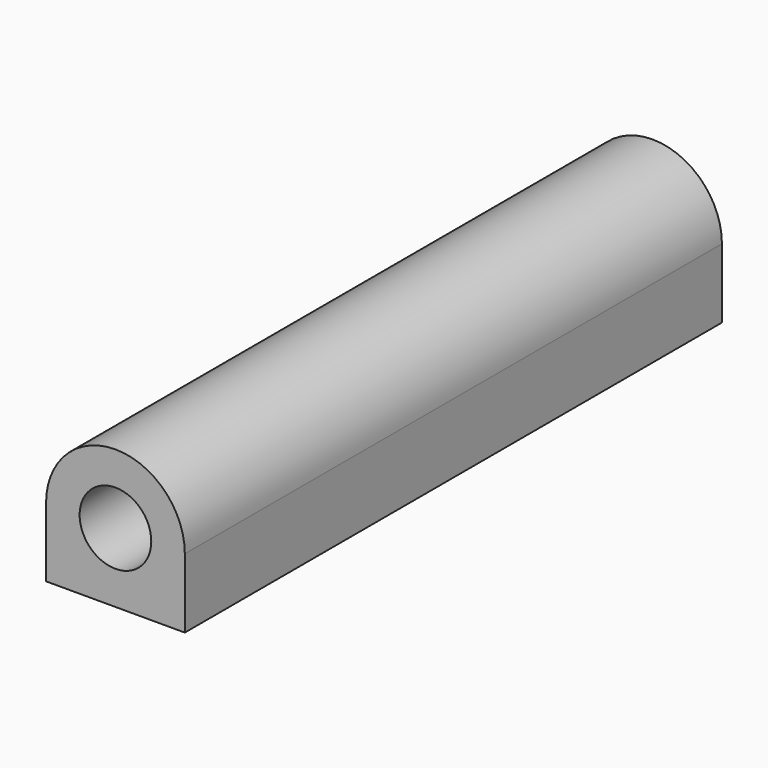
from build123d import *

# Parameters (mm, degrees)
F0_R         = 3.2
F1_DEPTH     = 30
F2_TEXT_SIZE = 11.1111111111
F3_DEPTH     = 0.6
F4_R         = 3.2
F5_DEPTH     = 2


# Not quite as in the source:
# - Text() gives the source's letters only with a copy of the font that has no kerning and outlines rounded to 1/6400 em; it was checked with that copy


with BuildPart() as f1:
    # F0 (on Front) → F1 (new body, symmetric)
    with BuildSketch(Plane.XZ):
        with BuildLine():
            ThreePointArc((0, -6.2), (4.3840620434, -4.3840620434), (6.2, 0))
            ThreePointArc((6.2, 0), (0, 6.2), (-6.2, 0))
            ThreePointArc((-6.2, 0), (-4.3840620434, -4.3840620434), (0, -6.2))
        make_face()
        Circle(F0_R, mode=Mode.SUBTRACT)
        with BuildLine():
            Line((6.2, -6.2), (6.2, 0))
            ThreePointArc((6.2, 0), (4.3840620434, -4.3840620434), (0, -6.2))
            Line((0, -6.2), (6.2, -6.2))
        make_face()
        with BuildLine():
            ThreePointArc((0, -6.2), (-4.3840620434, -4.3840620434), (-6.2, 0))
            Line((-6.2, 0), (-6.2, -6.2))
            Line((-6.2, -6.2), (0, -6.2))
        make_face()
    extrude(amount=F1_DEPTH, both=True)

    # F2 (on face) → F3 (cut)
    with BuildSketch(Plane(origin=(0, 0, -6.2), x_dir=(1, 0, 0), z_dir=(0, 0, -1))):
        with BuildLine():
            Line((1.6892361111, 11.2586805556), (1.1892361111, 11.2586805556))
            Line((1.1892361111, 11.2586805556), (1.2118055556, 10.6180555556))
            add(Edge.make_bspline(
                [(1.2118055556, 10.6180555556), (1.2326388889, 9.8958333333), (1.4713541667, 9.5434027778)],
                knots=[0, 0, 0, 1, 1, 1], degree=2))
            add(Edge.make_bspline(
                [(1.4713541667, 9.5434027778), (1.7100694444, 9.1909722222), (2.1979166667, 9.1909722222)],
                knots=[0, 0, 0, 1, 1, 1], degree=2))
            add(Edge.make_bspline(
                [(2.1979166667, 9.1909722222), (2.8993055556, 9.1909722222), (2.8993055556, 9.9930555556)],
                knots=[0, 0, 0, 1, 1, 1], degree=2))
            add(Edge.make_bspline(
                [(2.8993055556, 9.9930555556), (2.8993055556, 10.5694444444), (2.5677083333, 10.9140625)],
                knots=[0, 0, 0, 1, 1, 1], degree=2))
            add(Edge.make_bspline(
                [(2.5677083333, 10.9140625), (2.2361111111, 11.2586805556), (1.6892361111, 11.2586805556)],
                knots=[0, 0, 0, 1, 1, 1], degree=2))
        make_face()
        with Locations(Location((4, -13.6215277778), (0, 0, 90))):
            Text('ilena', F2_TEXT_SIZE, font='Open Sans', font_style=FontStyle.BOLD, text_align=(TextAlign.LEFT, TextAlign.BOTTOM))
        with BuildLine():
            add(Edge.make_bspline(
                [(-0.6684027778, -2.625), (-1.0017361111, -2.9340277778), (-1.0017361111, -3.4600694444)],
                knots=[0, 0, 0, 1, 1, 1], degree=2))
            add(Edge.make_bspline(
                [(-1.0017361111, -3.4600694444), (-1.0017361111, -3.9861111111), (-0.6684027778, -4.2847222222)],
                knots=[0, 0, 0, 1, 1, 1], degree=2))
            add(Edge.make_bspline(
                [(-0.6684027778, -4.2847222222), (-0.3350694444, -4.5833333333), (0.2777777778, -4.6267361111)],
                knots=[0, 0, 0, 1, 1, 1], degree=2))
            Line((0.2777777778, -4.6267361111), (0.2777777778, -2.3038194444))
            add(Edge.make_bspline(
                [(0.2777777778, -2.3038194444), (-0.3350694444, -2.3159722222), (-0.6684027778, -2.625)],
                knots=[0, 0, 0, 1, 1, 1], degree=2))
        make_face()
    extrude(amount=-F3_DEPTH, mode=Mode.SUBTRACT)

    # F4 (on Front) → F5 (join, symmetric)
    with BuildSketch(Plane.XZ):
        Circle(F4_R)
    extrude(amount=F5_DEPTH, both=True)


solid = f1.part
